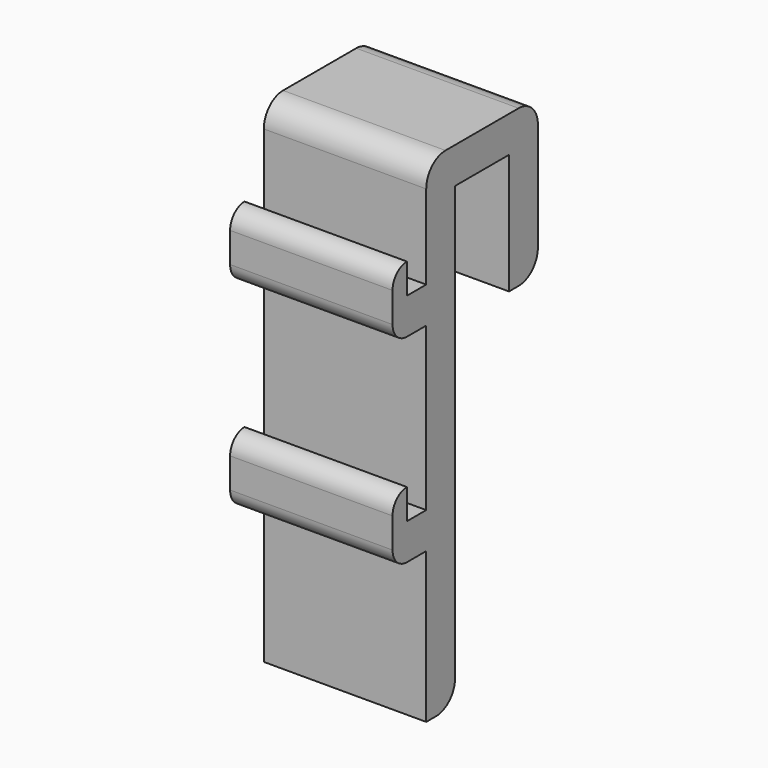
from build123d import *

# Parameters (mm, degrees)
F1_DEPTH = 13.5
F2_R     = 2
F3_R     = 1.49999
F4_ANGLE = 90
F5_ANGLE = 270


# Not quite as in the source:
# - a fillet or chamfer is up to 0.001 mm smaller than in the source, because OpenCascade refuses the exact size


with BuildPart() as f1:
    # F0 (on Top) → F1 (new body)
    with BuildSketch(Plane.XY):
        Polygon((0, 12.5), (0, 0), (3, 0), (3, 38), (8.6, 38), (8.6, 28), (11.6, 28), (11.6, 41), (0, 41), (0, 32), (-2, 32), (-2, 34.5), (-3.5, 34.5), (-3.5, 29), (0, 29), (0, 15.5), (-2, 15.5), (-2, 18), (-3.5, 18), (-3.5, 12.5), align=None)
    extrude(amount=F1_DEPTH)

    # F2
    f2_edges = [f1.edges().sort_by_distance(p)[0] for p in [
        (0, 41, 6.75),
        (11.6, 41, 6.75),
        (11.6, 28, 6.75),
        (3, 0, 6.75),
    ]]
    fillet(f2_edges, radius=F2_R)

    # F3 (radius 1.5 in the source; OpenCascade refuses exactly that, so slightly less here)
    f3_edges = [f1.edges().sort_by_distance(p)[0] for p in [
        (-3.5, 34.5, 6.75),
        (-3.5, 29, 6.75),
        (-3.5, 18, 6.75),
        (-3.5, 12.5, 6.75),
    ]]
    fillet(f3_edges, radius=F3_R)


with BuildPart() as f1_1:
    # F4: moved
    add(f1.part.rotate(Axis((0, 6.25, 13.5), (0, 1, 0)), F4_ANGLE))


with BuildPart() as f1_2:
    # F5: moved
    add(f1_1.part.rotate(Axis((-6.75, 0, 13.5), (-1, 0, 0)), F5_ANGLE))


solid = f1_2.part
